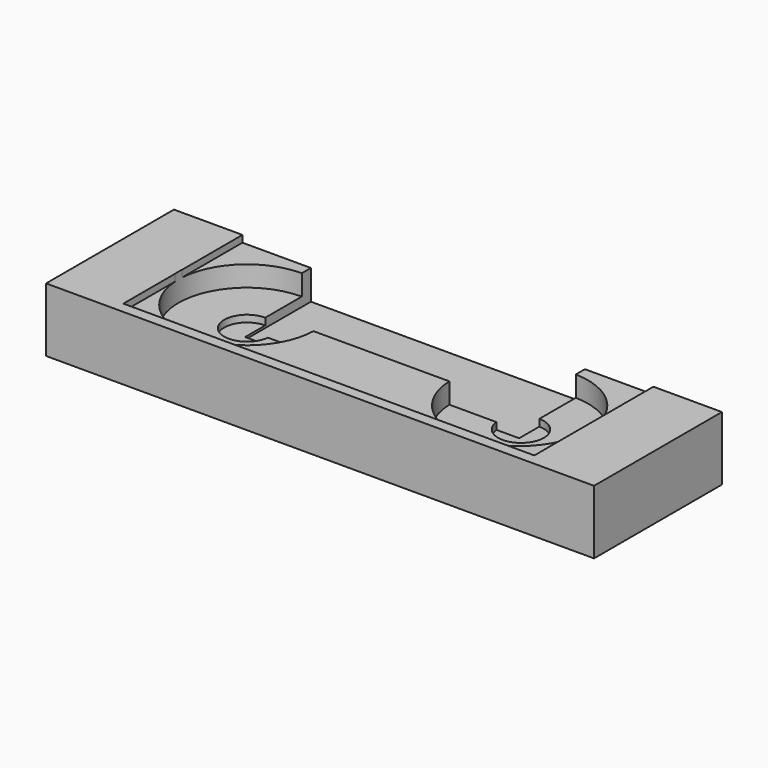
from build123d import *

# Parameters (mm, degrees)
F0_W      = 304.8
F0_H      = 88.9
F1_DEPTH  = 35.56
F2_R      = 38.1
F3_DEPTH  = 15.24
F4_R      = 38.1
F5_DEPTH  = 15.24
F6_W      = 152.4
F6_H      = 20.32
F7_DEPTH  = 45.72
F8_W      = 228.6
F8_H      = 82.7938915014
F9_DEPTH  = 3.81
F10_R     = 12.7
F11_DEPTH = 3.81
F12_R     = 12.7
F13_DEPTH = 3.81


# Not quite as in the source:
# - a feature of the source that left no trace in its solid (it failed there, or was rolled back) is left out


with BuildPart() as f1:
    # F0 (on Top) → F1 (new body)
    with BuildSketch(Plane.XY):
        Rectangle(F0_W, F0_H)
    extrude(amount=F1_DEPTH)

    # F2 (on face) → F3 (cut)
    with BuildSketch(Plane.XY.offset(35.56)):
        with Locations((75.4419565201, 0)):
            Circle(F2_R)
    extrude(amount=-F3_DEPTH, mode=Mode.SUBTRACT)

    # F4 (on face) → F5 (cut)
    with BuildSketch(Plane.XY.offset(35.56)):
        with Locations((-76.2725099921, 0)):
            Circle(F4_R)
    extrude(amount=-F5_DEPTH, mode=Mode.SUBTRACT)

    # F6 (on face) → F7 (cut)
    with BuildSketch(Plane(origin=(0, 44.45, 0), x_dir=(-1, 0, 0), z_dir=(0, 1, 0))):
        with Locations((0, 25.4)):
            Rectangle(F6_W, F6_H)
    extrude(amount=-F7_DEPTH, mode=Mode.SUBTRACT)

    # F8 (on face) → F9 (cut)
    with BuildSketch(Plane.XY.offset(35.56)):
        with Locations((0, 3.0530542493)):
            Rectangle(F8_W, F8_H)
    extrude(amount=-F9_DEPTH, mode=Mode.SUBTRACT)

    # F10 (on face) → F11 (cut)
    with BuildSketch(Plane.XY.offset(20.32)):
        with Locations((-76.2, 0)):
            Circle(F10_R)
    extrude(amount=-F11_DEPTH, mode=Mode.SUBTRACT)

    # F12 (on face) → F13 (cut)
    with BuildSketch(Plane.XY.offset(20.32)):
        with Locations((76.2, 0)):
            Circle(F12_R)
    extrude(amount=-F13_DEPTH, mode=Mode.SUBTRACT)


solid = f1.part
